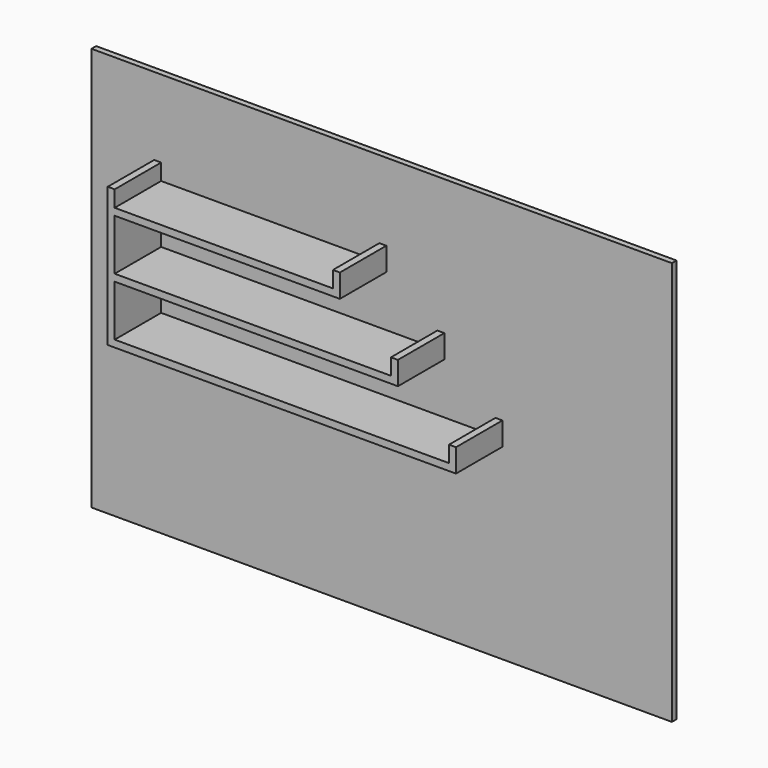
from build123d import *

# Parameters (mm, degrees)
F0_W     = 2500
F0_H     = 1739.7141116797
F1_DEPTH = 25
F3_W     = 30
F3_H     = 250


with BuildPart() as f1:
    # F0 (on Front) → F1 (new body)
    with BuildSketch(Plane.XZ):
        with Locations((965.0375247002, 49.0323135227)):
            Rectangle(F0_W, F0_H)
    extrude(amount=-F1_DEPTH)


with BuildPart() as f4:
    # F4: sweep along a path in F2
    with BuildLine(Plane.XZ) as f4_path:
        Line((1470, 85), (1470, 0))
        Line((1470, 0), (0, 0))
        Line((0, 0), (0, 250))
        Line((0, 250), (0, 500))
        Line((0, 500), (0, 585))
    # F3 (on Top) → F4 (sweep)
    with BuildSketch(Plane.XY):
        with Locations((0, -125)):
            Rectangle(F3_W, F3_H)
    sweep(path=f4_path.line, transition=Transition.RIGHT)

    # F5: sweep along a path in F2
    with BuildLine(Plane.XZ) as f5_path:
        Line((0, 0), (0, 250))
        Line((0, 250), (1220, 250))
        Line((1220, 250), (1220, 335))
    # F3 (on Top) → F5 (sweep)
    with BuildSketch(Plane.XY):
        with Locations((0, -125)):
            Rectangle(F3_W, F3_H)
    sweep(path=f5_path.line, transition=Transition.RIGHT)

    # F6: sweep along a path in F2
    with BuildLine(Plane.XZ) as f6_path:
        Line((0, 0), (0, 250))
        Line((0, 250), (0, 500))
        Line((0, 500), (970, 500))
        Line((970, 500), (970, 585))
    # F3 (on Top) → F6 (sweep)
    with BuildSketch(Plane.XY):
        with Locations((0, -125)):
            Rectangle(F3_W, F3_H)
    sweep(path=f6_path.line, transition=Transition.RIGHT)


solid = Compound([f1.part, f4.part])
